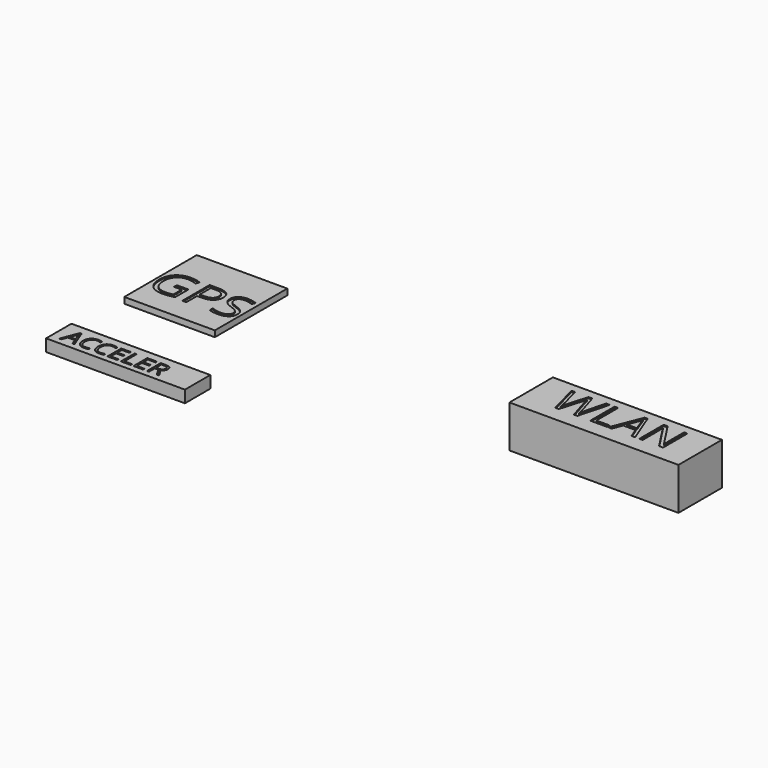
from build123d import *

# Parameters (mm, degrees)
F0_W          = 19.05
F0_H          = 19.05
F1_DEPTH      = 1.27
F2_TEXT_SIZE  = 10.0486277096
F3_DEPTH      = 0.254
F4_W          = 35.56
F4_H          = 11.43
F5_DEPTH      = 8.89
F6_TEXT_SIZE  = 8.9644247459
F7_DEPTH      = 0.254
F8_W          = 29.21
F8_H          = 6.6716015208
F9_DEPTH      = 2.54
F10_TEXT_SIZE = 5.0928029749
F11_DEPTH     = 1.27


# Not quite as in the source:
# - Text() gives the source's letters only with a copy of the font that has no kerning and outlines rounded to 1/6400 em; it was checked with that copy


with BuildPart() as f1:
    # F0 (on Top) → F1 (new body)
    with BuildSketch(Plane.XY):
        with Locations((-47.0747631265, -39.2846968025)):
            Rectangle(F0_W, F0_H)
    extrude(amount=F1_DEPTH)

    # F2 (on face) → F3 (cut)
    with BuildSketch(Plane.XY.offset(1.27)):
        with Locations((-56.5997631265, -43.918066636)):
            Text('GPS', F2_TEXT_SIZE, font='Open Sans', text_align=(TextAlign.LEFT, TextAlign.BOTTOM))
    extrude(amount=-F3_DEPTH, mode=Mode.SUBTRACT)


with BuildPart() as f5:
    # F4 (on Top) → F5 (new body)
    with BuildSketch(Plane.XY):
        with Locations((43.177546002, -44.3215195915)):
            Rectangle(F4_W, F4_H)
    extrude(amount=F5_DEPTH)

    # F6 (on face) → F7 (cut)
    with BuildSketch(Plane.XY.offset(8.89)):
        with Locations((30.6350551602, -46.8053035438)):
            Text('WLAN', F6_TEXT_SIZE, font='Open Sans', text_align=(TextAlign.LEFT, TextAlign.BOTTOM))
    extrude(amount=-F7_DEPTH, mode=Mode.SUBTRACT)


with BuildPart() as f9:
    # F8 (on Top) → F9 (new body)
    with BuildSketch(Plane.XY):
        with Locations((-41.2999819964, -66.9047795236)):
            Rectangle(F8_W, F8_H)
    extrude(amount=F9_DEPTH)

    # F10 (on face) → F11 (cut)
    with BuildSketch(Plane.XY.offset(2.54)):
        with Locations((-54.1608855128, -68.9698383212)):
            Text('ACCELER', F10_TEXT_SIZE, font='Open Sans', text_align=(TextAlign.LEFT, TextAlign.BOTTOM))
    extrude(amount=-F11_DEPTH, mode=Mode.SUBTRACT)


solid = Compound([f1.part, f5.part, f9.part])
